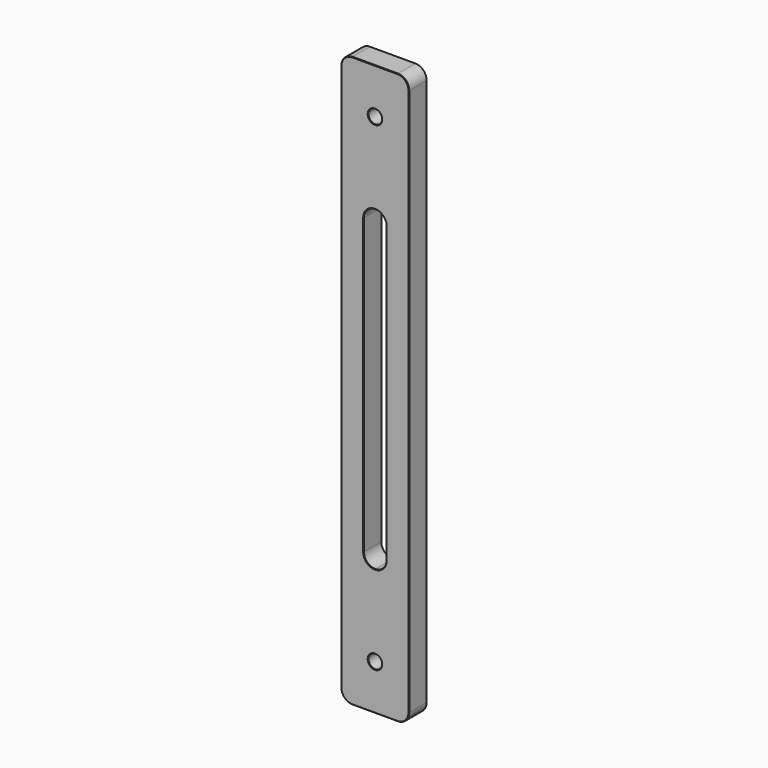
from build123d import *

# Parameters (mm, degrees)
F0_W     = 30
F0_H     = 252
F1_DEPTH = 10
F2_R     = 5
F4_DEPTH = 25
F5_R     = 4.99999
F6_R     = 3
F7_DEPTH = 25
F8_R     = 3
F9_DEPTH = 25
F10_SIZE = 0.2
F11_SIZE = 0.2


# Not quite as in the source:
# - a fillet or chamfer is up to 0.001 mm smaller than in the source, because OpenCascade refuses the exact size


with BuildPart() as f1:
    # F0 (on Front) → F1 (new body)
    with BuildSketch(Plane.XZ):
        with Locations((15, 126)):
            Rectangle(F0_W, F0_H)
    extrude(amount=F1_DEPTH)

    # F2
    f2_edges = [f1.edges().sort_by_distance(p)[0] for p in [
        (30, -5, 252),
        (0, -5, 252),
        (30, -5, 0),
        (0, -5, 0),
    ]]
    fillet(f2_edges, radius=F2_R)

    # F3 (on face) → F4 (cut)
    with BuildSketch(Plane.XZ.offset(10)):
        Polygon((10.0000001118, 196), (10.0000001118, 126), (10.0000001118, 56), (20, 56), (20, 126), (20, 196), align=None)
    extrude(amount=-F4_DEPTH, mode=Mode.SUBTRACT)

    # F5 (radius 5 in the source; OpenCascade refuses exactly that, so slightly less here)
    f5_edges = [f1.edges().sort_by_distance(p)[0] for p in [
        (10, -5, 196),
        (20, -5, 196),
        (20, -5, 56),
        (10, -5, 56),
    ]]
    fillet(f5_edges, radius=F5_R)

    # F6 (on face) → F7 (cut)
    with BuildSketch(Plane.XZ.offset(10)):
        with Locations((15, 232)):
            Circle(F6_R)
    extrude(amount=-F7_DEPTH, mode=Mode.SUBTRACT)

    # F8 (on face) → F9 (cut)
    with BuildSketch(Plane.XZ.offset(10)):
        with Locations((15, 20)):
            Circle(F8_R)
    extrude(amount=-F9_DEPTH, mode=Mode.SUBTRACT)

    # F10
    f10_edges = [f1.edges().sort_by_distance(p)[0] for p in [
        (0, -10, 126),
        (1.464466, -10, 250.535534),
        (1.464466, -10, 1.464466),
        (15, -10, 252),
        (15, -10, 0),
        (28.535534, -10, 250.535534),
        (28.535534, -10, 1.464466),
        (30, -10, 126),
        (12, -10, 20),
        (12, -10, 232),
        (15, -10, 56),
        (11.464463, -10, 57.464463),
        (18.535537, -10, 57.464463),
        (10, -10, 126),
        (20, -10, 126),
        (11.464463, -10, 194.535537),
        (18.535537, -10, 194.535537),
        (15, -10, 196),
    ]]
    chamfer(f10_edges, length=F10_SIZE)

    # F11
    f11_edges = [f1.edges().sort_by_distance(p)[0] for p in [
        (0, 0, 126),
        (1.464466, 0, 250.535534),
        (1.464466, 0, 1.464466),
        (15, 0, 252),
        (15, 0, 0),
        (28.535534, 0, 250.535534),
        (28.535534, 0, 1.464466),
        (30, 0, 126),
        (12, 0, 20),
        (12, 0, 232),
        (10, 0, 126),
        (11.464463, 0, 194.535537),
        (11.464463, 0, 57.464463),
        (15, 0, 196),
        (15, 0, 56),
        (18.535537, 0, 194.535537),
        (18.535537, 0, 57.464463),
        (20, 0, 126),
    ]]
    chamfer(f11_edges, length=F11_SIZE)


solid = f1.part
